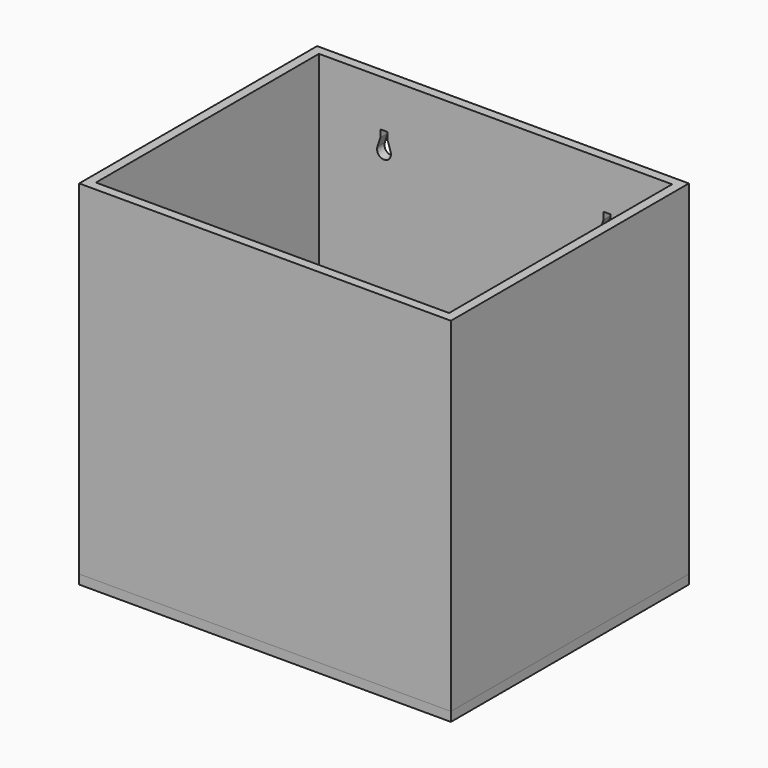
from build123d import *

# Parameters (mm, degrees)
F0_W     = 254
F0_H     = 203.2
F0_W_2   = 241.3
F0_H_2   = 190.5
F1_DEPTH = 234.95
F2_DEPTH = 6.35
F4_DEPTH = 12.7


# Not quite as in the source:
# - a feature of the source that left no trace in its solid (it failed there, or was rolled back) is left out


with BuildPart() as f1:
    # F0 (on Top) → F1 (new body)
    with BuildSketch(Plane.XY):
        Rectangle(F0_W, F0_H)
        Rectangle(F0_W_2, F0_H_2, mode=Mode.SUBTRACT)
    extrude(amount=F1_DEPTH)

    # F3 (on face) → F4 (cut)
    with BuildSketch(Plane(origin=(0, 101.6, 0), x_dir=(-1, 0, 0), z_dir=(0, 1, 0))):
        with BuildLine():
            ThreePointArc((-80.7195704438, 192.0016288669), (-76.2, 185.7375), (-71.6804295562, 192.0016288669))
            Line((-71.6804295562, 192.0016288669), (-73.81875, 198.4375))
            Line((-73.81875, 198.4375), (-73.81875, 203.2))
            Line((-73.81875, 203.2), (-78.58125, 203.2))
            Line((-78.58125, 203.2), (-78.58125, 198.4375))
            Line((-78.58125, 198.4375), (-80.7195704438, 192.0016288669))
        make_face()
        with BuildLine():
            Line((73.81875, 198.4375), (71.6804295562, 192.0016288669))
            ThreePointArc((71.6804295562, 192.0016288669), (76.2, 185.7375), (80.7195704438, 192.0016288669))
            Line((80.7195704438, 192.0016288669), (78.58125, 198.4375))
            Line((78.58125, 198.4375), (78.58125, 203.2))
            Line((78.58125, 203.2), (73.81875, 203.2))
            Line((73.81875, 203.2), (73.81875, 198.4375))
        make_face()
    extrude(amount=-F4_DEPTH, mode=Mode.SUBTRACT)


with BuildPart() as f2:
    # F0 (on Top) → F2 (new body)
    with BuildSketch(Plane.XY):
        Rectangle(F0_W, F0_H)
        Rectangle(F0_W_2, F0_H_2, mode=Mode.SUBTRACT)
        Rectangle(F0_W_2, F0_H_2)
    extrude(amount=-F2_DEPTH)


solid = Compound([f1.part, f2.part])
